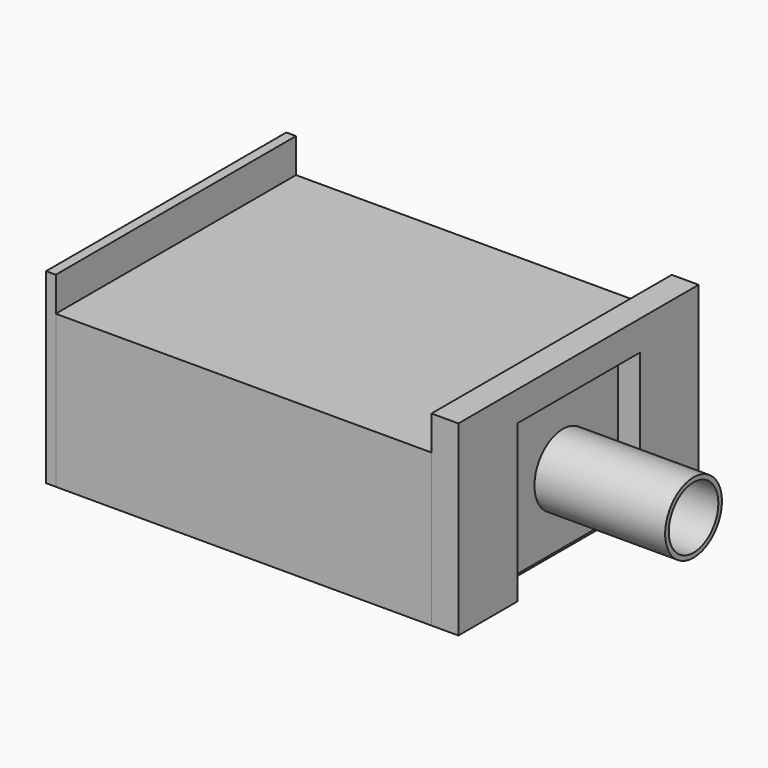
from build123d import *

# Parameters (mm, degrees)
F0_W     = 50.3
F0_H     = 20.4
F1_DEPTH = 20.1
F2_R     = 4.75
F3_DEPTH = 1.5
F4_DEPTH = 19
F5_T     = -0.6
F6_W     = 3.6
F6_H     = 40.2
F7_DEPTH = 25
F6_W_2   = 1.3
F9_DEPTH = 3.6


# Not quite as in the source:
# - a feature of the source that left no trace in its solid (it failed there, or was rolled back) is left out


with BuildPart() as f1:
    # F0 (on Front) → F1 (new body, symmetric)
    with BuildSketch(Plane.XZ):
        with Locations((2.45, 10.2)):
            Rectangle(F0_W, F0_H)
    extrude(amount=F1_DEPTH, both=True)

    # F2 (on face) → F3 (join)
    with BuildSketch(Plane.YZ.offset(27.6)):
        Polygon((-9.25, 20), (-9.25, 1.5), (0, 1.5), (9.25, 1.5), (9.25, 20), (0, 20), align=None)
        with Locations((0, 10.75)):
            Circle(F2_R, mode=Mode.SUBTRACT)
    extrude(amount=F3_DEPTH)

    # F4 (add): a face of the model
    f4_faces = [f1.faces().sort_by_distance(p)[0] for p in [
        (27.6, 0, 10.75),
    ]]
    extrude(f4_faces, amount=F4_DEPTH)

    # F5
    f5_openings = [f1.faces().sort_by_distance(p)[0] for p in [
        (46.6, 0, 10.75),
    ]]
    offset(amount=F5_T, openings=f5_openings, kind=Kind.INTERSECTION)


with BuildPart() as f7:
    # F6 (on Top) → F7 (new body)
    with BuildSketch(Plane.XY):
        with Locations((29.4, 0)):
            Rectangle(F6_W, F6_H)
    extrude(amount=F7_DEPTH)

    # F8 (on face) → F9 (cut, through all)
    with BuildSketch(Plane.YZ.offset(31.2)):
        with BuildLine():
            Line((-9.25, 0), (-9.25, 16.108633541))
            ThreePointArc((-9.25, 16.108633541), (-9.7456992731, 16.015473058), (-10.25, 16.0066740906))
            Line((-10.25, 16.0066740906), (-10.25, 0))
            Line((-10.25, 0), (-9.25, 0))
        make_face()
        with BuildLine():
            Line((-9.25, 16.108633541), (-9.25, 20))
            Line((-9.25, 20), (-7.2215728753, 20))
            ThreePointArc((-7.2215728753, 20), (-7.4688611699, 20.5289611963), (-7.8139320225, 21))
            Line((-7.8139320225, 21), (-10.25, 21))
            Line((-10.25, 21), (-10.25, 16.0066740906))
            ThreePointArc((-10.25, 16.0066740906), (-9.7456992731, 16.015473058), (-9.25, 16.108633541))
        make_face()
        with BuildLine():
            ThreePointArc((-7.8139320225, 21), (-7.4688611699, 20.5289611963), (-7.2215728753, 20))
            Line((-7.2215728753, 20), (-2.8284271247, 20))
            ThreePointArc((-2.8284271247, 20), (-2.5811388301, 20.5289611963), (-2.2360679775, 21))
            Line((-2.2360679775, 21), (-7.8139320225, 21))
        make_face()
        with BuildLine():
            Line((-2.8284271247, 20), (-7.2215728753, 20))
            ThreePointArc((-7.2215728753, 20), (-7.093204321, 19.5073059362), (-7.05, 19))
            ThreePointArc((-7.05, 19), (-7.6625327227, 17.1834097875), (-9.25, 16.108633541))
            Line((-9.25, 16.108633541), (-9.25, 0))
            Line((-9.25, 0), (9.25, 0))
            Line((9.25, 0), (9.25, 16.108633541))
            ThreePointArc((9.25, 16.108633541), (7.3897266908, 17.6132967438), (7.2215728753, 20))
            Line((7.2215728753, 20), (2.8284271247, 20))
            ThreePointArc((2.8284271247, 20), (2.956795679, 19.5073059362), (3, 19))
            ThreePointArc((3, 19), (-0.5073059362, 16.043204321), (-2.8284271247, 20))
        make_face()
        with BuildLine():
            Line((9.25, 20), (7.2215728753, 20))
            ThreePointArc((7.2215728753, 20), (7.3897266908, 17.6132967438), (9.25, 16.108633541))
            Line((9.25, 16.108633541), (9.25, 20))
        make_face()
        with BuildLine():
            Line((2.8284271247, 20), (-2.8284271247, 20))
            ThreePointArc((-2.8284271247, 20), (-0.5073059362, 16.043204321), (3, 19))
            ThreePointArc((3, 19), (2.956795679, 19.5073059362), (2.8284271247, 20))
        make_face()
        with BuildLine():
            Line((-7.2215728753, 20), (-9.25, 20))
            Line((-9.25, 20), (-9.25, 16.108633541))
            ThreePointArc((-9.25, 16.108633541), (-7.6625327227, 17.1834097875), (-7.05, 19))
            ThreePointArc((-7.05, 19), (-7.093204321, 19.5073059362), (-7.2215728753, 20))
        make_face()
        with BuildLine():
            Line((9.25, 16.108633541), (9.25, 0))
            Line((9.25, 0), (10.25, 0))
            Line((10.25, 0), (10.25, 16.0066740906))
            ThreePointArc((10.25, 16.0066740906), (9.7456992731, 16.015473058), (9.25, 16.108633541))
        make_face()
        with BuildLine():
            ThreePointArc((7.8139320225, 21), (7.4688611699, 20.5289611963), (7.2215728753, 20))
            Line((7.2215728753, 20), (9.25, 20))
            Line((9.25, 20), (9.25, 16.108633541))
            ThreePointArc((9.25, 16.108633541), (9.7456992731, 16.015473058), (10.25, 16.0066740906))
            Line((10.25, 16.0066740906), (10.25, 21))
            Line((10.25, 21), (7.8139320225, 21))
        make_face()
        with BuildLine():
            ThreePointArc((2.2360679775, 21), (2.5811388301, 20.5289611963), (2.8284271247, 20))
            Line((2.8284271247, 20), (7.2215728753, 20))
            ThreePointArc((7.2215728753, 20), (7.4688611699, 20.5289611963), (7.8139320225, 21))
            Line((7.8139320225, 21), (2.2360679775, 21))
        make_face()
        with BuildLine():
            ThreePointArc((-2.2360679775, 21), (-2.5811388301, 20.5289611963), (-2.8284271247, 20))
            Line((-2.8284271247, 20), (2.8284271247, 20))
            ThreePointArc((2.8284271247, 20), (2.5811388301, 20.5289611963), (2.2360679775, 21))
            Line((2.2360679775, 21), (-2.2360679775, 21))
        make_face()
    extrude(amount=-F9_DEPTH, mode=Mode.SUBTRACT)


with BuildPart() as f7b:
    # F6 (on Top) → F7, piece 2 (new body)
    with BuildSketch(Plane.XY):
        with Locations((-23.35, 0)):
            Rectangle(F6_W_2, F6_H)
    extrude(amount=F7_DEPTH)


solid = Compound([f1.part, f7.part, f7b.part])
